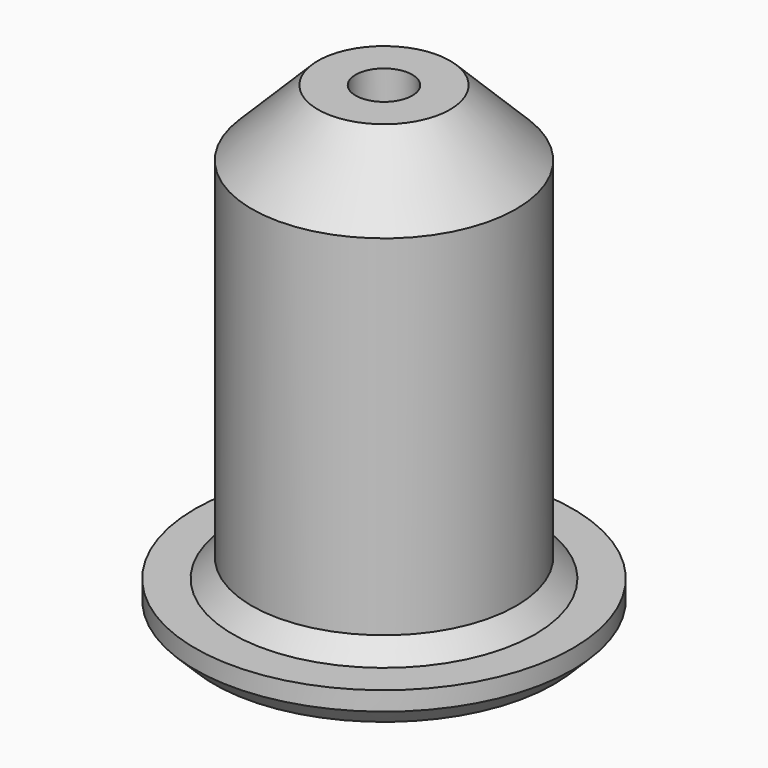
from build123d import *

# Parameters (mm, degrees)
F0_R     = 7
F0_R_2   = 1.5
F1_DEPTH = 25
F2_T     = -2
F3_DEPTH = 25
F4_R     = 10
F4_R_2   = 7
F5_DEPTH = 2
F6_SIZE  = 1
F7_SIZE  = 3.49999


# Not quite as in the source:
# - a fillet or chamfer is up to 0.001 mm smaller than in the source, because OpenCascade refuses the exact size


with BuildPart() as f1:
    # F0 (on Top) → F1 (new body)
    with BuildSketch(Plane.XY):
        Circle(F0_R)
        Circle(F0_R_2, mode=Mode.SUBTRACT)
        Circle(F0_R_2)
    extrude(amount=-F1_DEPTH)

    # F2
    f2_openings = [f1.faces().sort_by_distance(p)[0] for p in [
        (0, 0, -25),
    ]]
    offset(amount=F2_T, openings=f2_openings)

    # F0 (on Top) → F3 (cut)
    with BuildSketch(Plane.XY):
        Circle(F0_R_2)
    extrude(amount=-F3_DEPTH, mode=Mode.SUBTRACT)

    # F4 (on face) → F5 (join)
    with BuildSketch(Plane(origin=(0, 0, -25), x_dir=(1, 0, 0), z_dir=(0, 0, -1))):
        Circle(F4_R)
        Circle(F4_R_2, mode=Mode.SUBTRACT)
    extrude(amount=-F5_DEPTH)

    # F6
    f6_edges = [f1.edges().sort_by_distance(p)[0] for p in [
        (-7, 0, -23),
        (-5, 0, -25),
        (-10, 0, -25),
    ]]
    chamfer(f6_edges, length=F6_SIZE)

    # F7 (size 3.5 in the source; OpenCascade refuses exactly that, so slightly less here)
    f7_edges = [f1.edges().sort_by_distance(p)[0] for p in [
        (-7, 0, 0),
        (-5, 0, -2),
    ]]
    chamfer(f7_edges, length=F7_SIZE)


solid = f1.part
